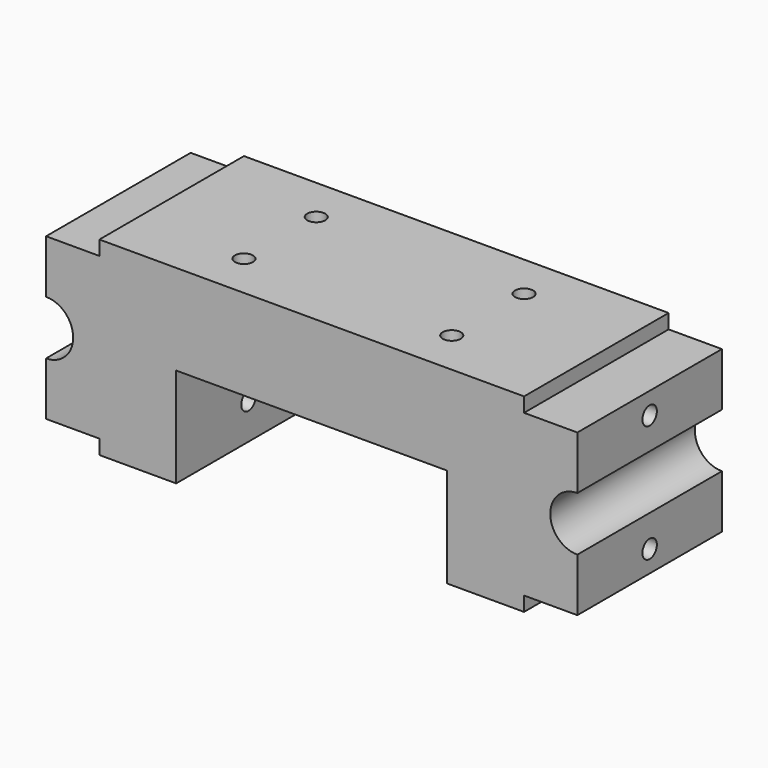
from build123d import *

# Parameters (mm, degrees)
F0_W      = 62
F0_H      = 53
F1_DEPTH  = 10
F3_DEPTH  = 20
F5_D      = 2
F6_W      = 9
F6_H      = 4.25
F7_DEPTH  = 20
F8_W      = 57.8
F8_H      = 29.9
F9_DEPTH  = 25
F10_W     = 30
F10_H     = 20
F11_DEPTH = 11
F13_D     = 2
F13_DEPTH = 80
F13_TIP   = 0.600860619
F14_R     = 3
F15_DEPTH = 25


# Not quite as in the source:
# - a pattern or mirror of a feature is missing from the dataset's text; its kind, count and spacing are read off the source's solid


with BuildPart() as f1:
    # F0 (on Front) → F1 (new body, symmetric)
    with BuildSketch(Plane.XZ):
        Rectangle(F0_W, F0_H)
    extrude(amount=F1_DEPTH, both=True)

    # F2 (on face) → F3 (cut, through all)
    with BuildSketch(Plane.XZ.offset(10)):
        Polygon((-16, 26.5), (-31, 26.5), (-31, -5.5), (-28.9, -5.5), (-28.9, 24.4), (-16, 24.4), align=None)
        Polygon((-28.9, -5.5), (-31, -5.5), (-31, -26.5), (-23.5, -26.5), (-23.5, -24.9), (-29.4, -24.9), (-29.4, -7.1), (-23.5, -7.1), (-23.5, -5.5), align=None)
    f3 = extrude(amount=-F3_DEPTH, mode=Mode.SUBTRACT)

    # F3_copies: F3 across plane
    add(f3.mirror(Plane(origin=(0, 0, 0), x_dir=(0, 0, 1), z_dir=(1, 0, 0))), mode=Mode.SUBTRACT)

    # F5 (through all)
    with Locations(Plane(origin=(-28.9, 0, 0), x_dir=(0, -1, 0), z_dir=(-1, 0, 0))):
        with Locations((0, 19), (0, 4), (0, -9.5), (0, -22.5)):
            Hole(F5_D / 2)

    # F6 (on face) → F7 (cut, through all)
    with BuildSketch(Plane.XZ.offset(10)):
        with Locations((-2.5, 24.375)):
            Rectangle(F6_W, F6_H)
        Polygon((-7, 22.25), (-7, 26.5), (-16, 26.5), (-16, 24.4), (-16, 22.25), align=None)
        with Locations((6.5, 24.375)):
            Rectangle(F6_W, F6_H)
        Polygon((16, 26.5), (11, 26.5), (11, 22.25), (16, 22.25), (16, 24.4), align=None)
    extrude(amount=-F7_DEPTH, mode=Mode.SUBTRACT)

    # F8 (on face) → F9 (cut)
    with BuildSketch(Plane.XZ.offset(10)):
        with Locations((0, 9.45)):
            Rectangle(F8_W, F8_H)
    extrude(amount=-F9_DEPTH, mode=Mode.SUBTRACT)

    # F10 (on face) → F11 (cut)
    with BuildSketch(Plane(origin=(0, 0, -26.5), x_dir=(1, 0, 0), z_dir=(0, 0, -1))):
        Rectangle(F10_W, F10_H)
    extrude(amount=-F11_DEPTH, mode=Mode.SUBTRACT)

    # F13
    with Locations(Plane(origin=(0, 0, -15.5), x_dir=(1, 0, 0), z_dir=(0, 0, -1))):
        with Locations((-11.5, 5), (11.5, 5), (11.5, -5), (-11.5, -5)):
            Hole(F13_D / 2, depth=F13_DEPTH)
            with Locations((0, 0, -(F13_DEPTH + F13_TIP / 2))):  # 118° drill point
                Cone(0, F13_D / 2, F13_TIP, mode=Mode.SUBTRACT)

    # F14 (on face) → F15 (cut)
    with BuildSketch(Plane.XZ.offset(10)):
        with Locations((-29.4, -16)):
            Circle(F14_R)
        with Locations((29.4, -16)):
            Circle(F14_R)
    extrude(amount=-F15_DEPTH, mode=Mode.SUBTRACT)


solid = f1.part
